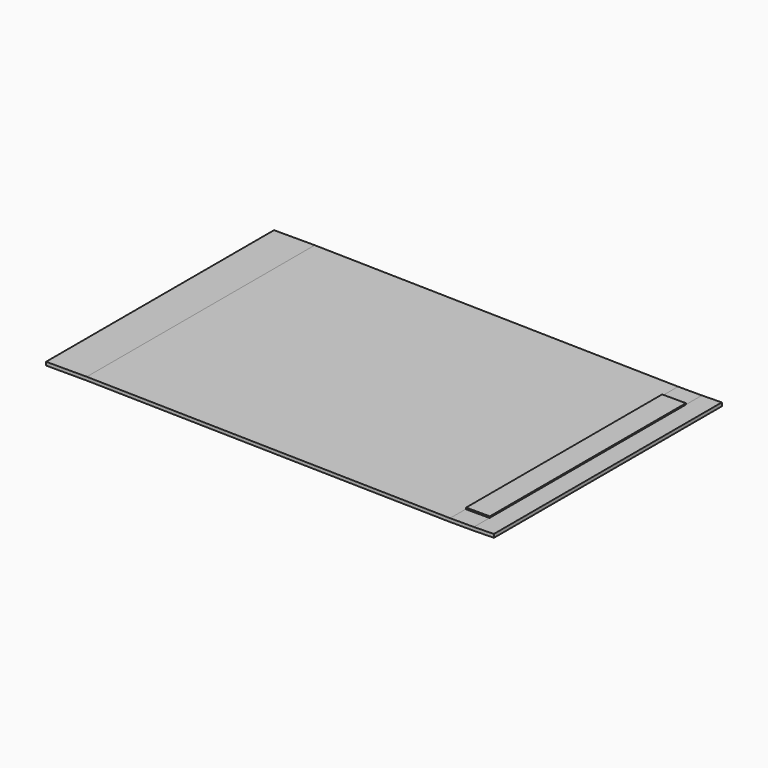
from build123d import *

# Parameters (mm, degrees)
F0_W           = 85.725
F0_H           = 914.4
F0_R           = 25.4
F0_R_2         = 22.225
F1_DEPTH       = 38.1
F2_DEPTH       = 76.2
F4_DEPTH       = 85.726
F5_W           = 88.9
F5_H           = 917.575
F5_W_2         = 85.725
F5_H_2         = 914.4
F6_DEPTH       = 6.35
F10_DEPTH      = 533.4
F10_DEPTH_BACK = 533.4
F11_W          = 89.1216455618
F11_H          = 920.75
F12_DEPTH      = 71.4394671358


# Not quite as in the source:
# - a length typed as a fraction of an inch, garbled in the dataset ("3 / 203.2 mm" for 3/8 in), is restored
# - a pattern or mirror of a feature is missing from the dataset's text; its kind, count and spacing are read off the source's solid


with BuildPart() as f1:
    # F0 (on Top) → F1 (new body)
    with BuildSketch(Plane.XY):
        Rectangle(F0_W, F0_H)
        Circle(F0_R, mode=Mode.SUBTRACT)
        Circle(F0_R)
        Circle(F0_R_2, mode=Mode.SUBTRACT)
        Circle(F0_R_2)
    extrude(amount=-F1_DEPTH)



with BuildPart() as f2:
    # F0 (on Top) → F2 (new body)
    with BuildSketch(Plane.XY):
        Circle(F0_R_2)
    extrude(amount=-F2_DEPTH)


with BuildPart() as f1_1:
    add(f1.part)

    add(f2.part)  # F2_copies merges F2
    # F2_copies: F2 across plane
    add(f2.part.mirror(Plane(origin=(0, 0, -38.1), x_dir=(-1, 0, 0), z_dir=(0, 0, -1))))

    # F3 (on face) → F4 (cut, through all)
    with BuildSketch(Plane.YZ.offset(42.8625)):
        Polygon((-457.2, -38.1), (0, -38.1), (-457.2, -19.05), align=None)
        Polygon((457.2, -19.05), (0, -38.1), (457.2, -38.1), align=None)
    extrude(amount=-F4_DEPTH, mode=Mode.SUBTRACT)


with BuildPart() as f6:
    # F5 (on face) → F6 (new body)
    with BuildSketch(Plane.XY):
        Rectangle(F5_W, F5_H)
        Rectangle(F5_W_2, F5_H_2, mode=Mode.SUBTRACT)
    extrude(amount=-F6_DEPTH)


with BuildPart() as f10:
    # F9 (on Front) → F10 (new body, two sides)
    with BuildSketch(Plane.XZ) as f10_sk:
        Polygon((119.207431633, -3.4585714601), (44.5608227809, -4.7615328642), (45.0041139044, -17.4557297551), (119.6507227565, -16.1527683509), align=None)
        Polygon((-44.7824683426, -17.4595985927), (-44.5608227809, -4.7615328642), (-1404.9375, 18.9839303634), (-1404.9375, 6.285864635), (-1405.1591455618, 6.285864635), align=None)
        Polygon((-1404.9375, 6.285864635), (-1404.9375, 18.9839303634), (-1557.3375, 18.9839303634), (-1557.3375, 6.285864635), (-1405.1591455618, 6.285864635), align=None)
        Polygon((44.5608227809, -4.7615328642), (-44.5608227809, -4.7615328642), (-44.7824683426, -17.4595985927), (45.0041139044, -17.4557297551), align=None)
    extrude(amount=F10_DEPTH)
    extrude(f10_sk.sketch, amount=-F10_DEPTH_BACK)

    # F11 (on face) → F12 (cut, through all)
    with BuildSketch(Plane.XY.offset(-4.7615328642)):
        Rectangle(F11_W, F11_H)
    extrude(amount=-F12_DEPTH, mode=Mode.SUBTRACT)


solid = Compound([f1_1.part, f6.part, f10.part])
